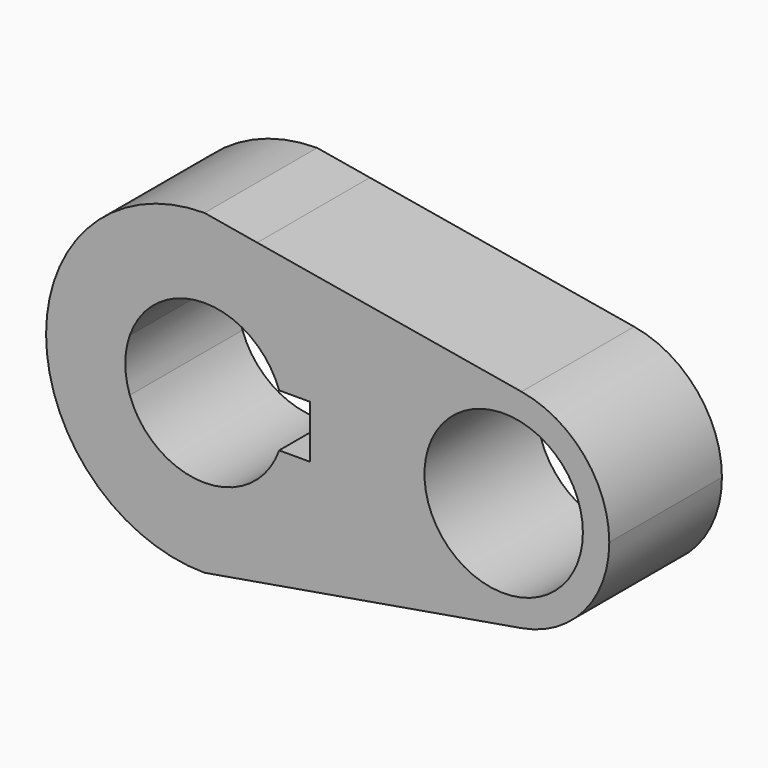
from build123d import *

# Parameters (mm, degrees)
F0_R     = 14.2875
F1_DEPTH = 25.4


with BuildPart() as f1:
    # F0 (on Front) → F1 (new body)
    with BuildSketch(Plane.XZ):
        with BuildLine():
            Line((9.5121844836, 26.9452959039), (0, 28.575))
            ThreePointArc((0, 28.575), (-28.575, 0), (0, -28.575))
            Line((0, -28.575), (9.5121844836, -26.9452959039))
            ThreePointArc((9.5121844836, -26.9452959039), (23.3274655355, -16.5033322905), (28.575, 0))
            ThreePointArc((28.575, 0), (23.3274655355, 16.5033322905), (9.5121844836, 26.9452959039))
        make_face()
        with BuildLine():
            ThreePointArc((-13.4703841816, 4.7625), (0, 14.2875), (13.4703841816, 4.7625))
            Line((13.4703841816, 4.7625), (19.05, 4.7625))
            Line((19.05, 4.7625), (19.05, -4.7625))
            Line((19.05, -4.7625), (13.4703841816, -4.7625))
            ThreePointArc((13.4703841816, -4.7625), (0, -14.2875), (-13.4703841816, -4.7625))
            Line((-13.4703841816, -4.7625), (-19.05, -4.7625))
            Line((-19.05, -4.7625), (-19.05, 4.7625))
            Line((-19.05, 4.7625), (-13.4703841816, 4.7625))
        make_face(mode=Mode.SUBTRACT)
        with BuildLine():
            Line((57.1919272622, 18.7764181619), (9.5121844836, 26.9452959039))
            ThreePointArc((9.5121844836, 26.9452959039), (23.3274655355, 16.5033322905), (28.575, 0))
            ThreePointArc((28.575, 0), (23.3274655355, -16.5033322905), (9.5121844836, -26.9452959039))
            Line((9.5121844836, -26.9452959039), (57.1919272622, -18.7764181619))
            ThreePointArc((57.1919272622, -18.7764181619), (34.925, 0), (57.1919272622, 18.7764181619))
        make_face()
        with BuildLine():
            ThreePointArc((73.025, 0), (68.5383952831, 12.2804730295), (57.1919272622, 18.7764181619))
            ThreePointArc((57.1919272622, 18.7764181619), (34.925, 0), (57.1919272622, -18.7764181619))
            ThreePointArc((57.1919272622, -18.7764181619), (68.5383952831, -12.2804730295), (73.025, 0))
        make_face()
        with Locations((53.975, 0)):
            Circle(F0_R, mode=Mode.SUBTRACT)
        with BuildLine():
            ThreePointArc((-13.4703841816, -4.7625), (-14.2875, 0), (-13.4703841816, 4.7625))
            Line((-13.4703841816, 4.7625), (-19.05, 4.7625))
            Line((-19.05, 4.7625), (-19.05, -4.7625))
            Line((-19.05, -4.7625), (-13.4703841816, -4.7625))
        make_face()
    extrude(amount=F1_DEPTH)


solid = f1.part
